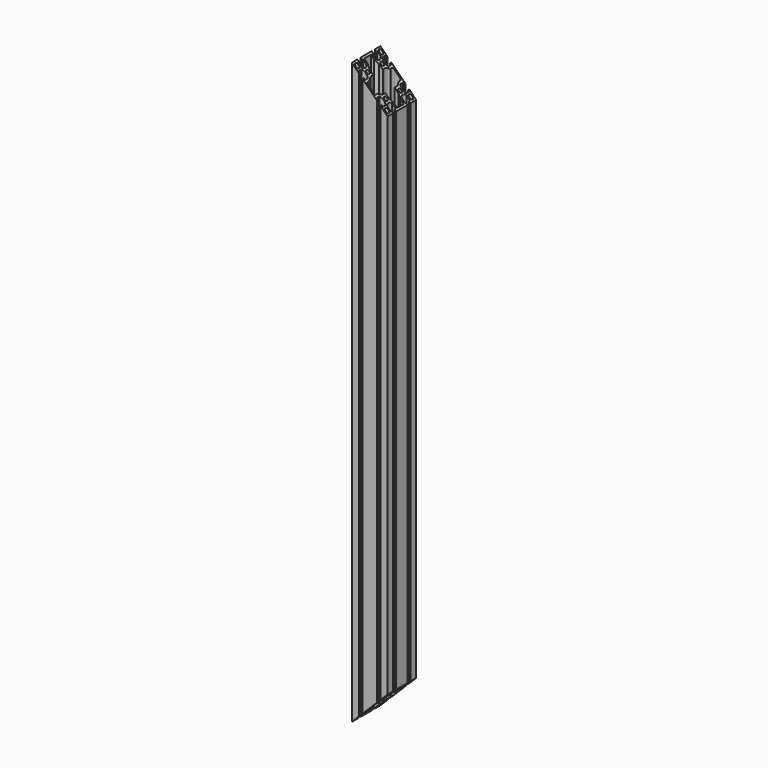
from build123d import *

# Parameters (mm, degrees)
F0_R     = 3
F0_R_2   = 2.5
F1_DEPTH = 973
F2_R     = 2
F3_R     = 7
F5_DEPTH = 60


# Not quite as in the source:
# - a feature names something its author has since deleted; it is built from what else it names


with BuildPart() as f1:
    # F0 (on Top) → F1 (new body)
    with BuildSketch(Plane.XY):
        with BuildLine():
            Line((18.15, -30), (30, -30))
            Line((30, -30), (30, -18.15))
            Line((30, -18.15), (27.5, -18.15))
            Line((27.5, -18.15), (27.5, -20.15))
            Line((27.5, -20.15), (21.5477069044, -20.15))
            ThreePointArc((21.5477069044, -20.15), (19.5, -15), (21.5477069044, -9.85))
            Line((21.5477069044, -9.85), (27.5, -9.85))
            Line((27.5, -9.85), (27.5, -11.85))
            Line((27.5, -11.85), (30, -11.85))
            Line((30, -11.85), (30, 11.85))
            Line((30, 11.85), (27.5, 11.85))
            Line((27.5, 11.85), (27.5, 9.85))
            Line((27.5, 9.85), (21.5477069044, 9.85))
            ThreePointArc((21.5477069044, 9.85), (19.5, 15), (21.5477069044, 20.15))
            Line((21.5477069044, 20.15), (27.5, 20.15))
            Line((27.5, 20.15), (27.5, 18.15))
            Line((27.5, 18.15), (30, 18.15))
            Line((30, 18.15), (30, 30))
            Line((30, 30), (18.15, 30))
            Line((18.15, 30), (18.15, 27.5))
            Line((18.15, 27.5), (20.15, 27.5))
            Line((20.15, 27.5), (20.15, 21.5477069044))
            ThreePointArc((20.15, 21.5477069044), (15, 19.5), (9.85, 21.5477069044))
            Line((9.85, 21.5477069044), (9.85, 27.5))
            Line((9.85, 27.5), (11.85, 27.5))
            Line((11.85, 27.5), (11.85, 30))
            Line((11.85, 30), (-11.85, 30))
            Line((-11.85, 30), (-11.85, 27.5))
            Line((-11.85, 27.5), (-9.85, 27.5))
            Line((-9.85, 27.5), (-9.85, 21.5477069044))
            ThreePointArc((-9.85, 21.5477069044), (-15, 19.5), (-20.15, 21.5477069044))
            Line((-20.15, 21.5477069044), (-20.15, 27.5))
            Line((-20.15, 27.5), (-18.15, 27.5))
            Line((-18.15, 27.5), (-18.15, 30))
            Line((-18.15, 30), (-30, 30))
            Line((-30, 30), (-30, 18.15))
            Line((-30, 18.15), (-27.5, 18.15))
            Line((-27.5, 18.15), (-27.5, 20.15))
            Line((-27.5, 20.15), (-21.5477069044, 20.15))
            ThreePointArc((-21.5477069044, 20.15), (-19.5, 15), (-21.5477069044, 9.85))
            Line((-21.5477069044, 9.85), (-27.5, 9.85))
            Line((-27.5, 9.85), (-27.5, 11.85))
            Line((-27.5, 11.85), (-30, 11.85))
            Line((-30, 11.85), (-30, -11.85))
            Line((-30, -11.85), (-27.5, -11.85))
            Line((-27.5, -11.85), (-27.5, -9.85))
            Line((-27.5, -9.85), (-21.5477069044, -9.85))
            ThreePointArc((-21.5477069044, -9.85), (-19.5, -15), (-21.5477069044, -20.15))
            Line((-21.5477069044, -20.15), (-27.5, -20.15))
            Line((-27.5, -20.15), (-27.5, -18.15))
            Line((-27.5, -18.15), (-30, -18.15))
            Line((-30, -18.15), (-30, -30))
            Line((-30, -30), (-18.15, -30))
            Line((-18.15, -30), (-18.15, -27.5))
            Line((-18.15, -27.5), (-20.15, -27.5))
            Line((-20.15, -27.5), (-20.15, -21.5477069044))
            ThreePointArc((-20.15, -21.5477069044), (-15, -19.5), (-9.85, -21.5477069044))
            Line((-9.85, -21.5477069044), (-9.85, -27.5))
            Line((-9.85, -27.5), (-11.85, -27.5))
            Line((-11.85, -27.5), (-11.85, -30))
            Line((-11.85, -30), (11.85, -30))
            Line((11.85, -30), (11.85, -27.5))
            Line((11.85, -27.5), (9.85, -27.5))
            Line((9.85, -27.5), (9.85, -21.5477069044))
            ThreePointArc((9.85, -21.5477069044), (15, -19.5), (20.15, -21.5477069044))
            Line((20.15, -21.5477069044), (20.15, -27.5))
            Line((20.15, -27.5), (18.15, -27.5))
            Line((18.15, -27.5), (18.15, -30))
        make_face()
        with Locations((-25, -25)):
            Circle(F0_R, mode=Mode.SUBTRACT)
        with Locations((-15, -15)):
            Circle(F0_R_2, mode=Mode.SUBTRACT)
        with Locations((25, -25)):
            Circle(F0_R, mode=Mode.SUBTRACT)
        with Locations((15, -15)):
            Circle(F0_R_2, mode=Mode.SUBTRACT)
        with Locations((-25, 25)):
            Circle(F0_R, mode=Mode.SUBTRACT)
        with Locations((-15, 15)):
            Circle(F0_R_2, mode=Mode.SUBTRACT)
        Polygon((-7, 22), (-7, 27.5), (0, 27.5), (7, 27.5), (7, 22), (10, 16), (10, 10), (16, 10), (22, 7), (27.5, 7), (27.5, 0), (27.5, -7), (22, -7), (16, -10), (10, -10), (10, -16), (7, -22), (7, -27.5), (0, -27.5), (-7, -27.5), (-7, -22), (-10, -16), (-10, -10), (-16, -10), (-22, -7), (-27.5, -7), (-27.5, 0), (-27.5, 7), (-22, 7), (-16, 10), (-10, 10), (-10, 16), align=None, mode=Mode.SUBTRACT)
        with Locations((15, 15)):
            Circle(F0_R_2, mode=Mode.SUBTRACT)
        with Locations((25, 25)):
            Circle(F0_R, mode=Mode.SUBTRACT)
    extrude(amount=F1_DEPTH)

    # F2
    f2_edges = [f1.edges().sort_by_distance(p)[0] for p in [
        (-7, 27.5, 486.5),
        (7, 27.5, 486.5),
    ]]
    fillet(f2_edges, radius=F2_R)

    # F3
    f3_edges = [f1.edges().sort_by_distance(p)[0] for p in [
        (-10, 16, 486.5),
        (10, 16, 486.5),
    ]]
    fillet(f3_edges, radius=F3_R)

    # F4 (on face) → F5 (cut)
    with BuildSketch(Plane.XZ.offset(30)):
        Polygon((30, 0), (30, 60), (-30, 0), (-18.15, 0), align=None)
        Polygon((30, 913), (30, 973), (-18.15, 973), (-30, 973), align=None)
    extrude(amount=-F5_DEPTH, mode=Mode.SUBTRACT)


solid = f1.part
